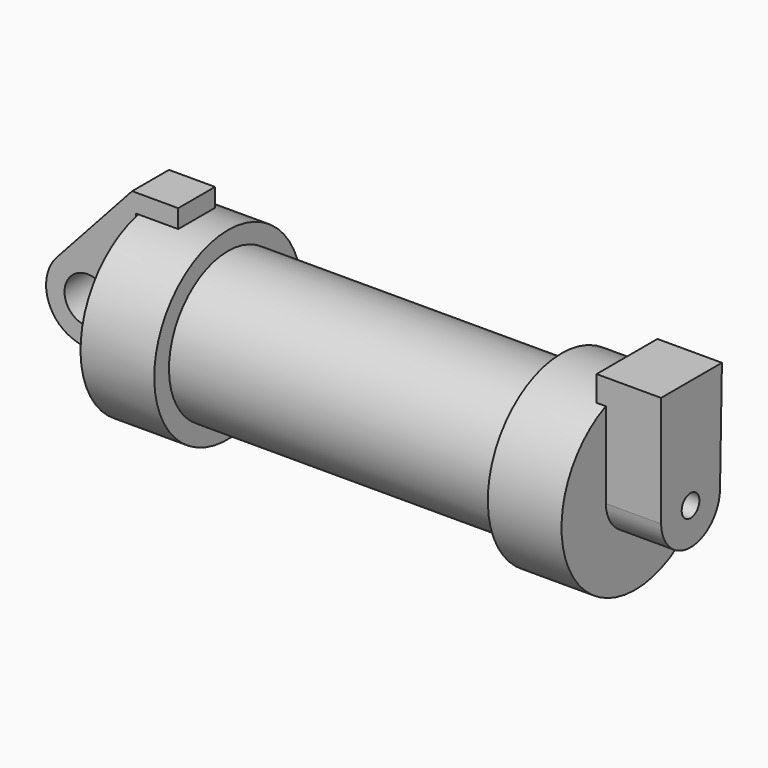
from build123d import *

# Parameters (mm, degrees)
F0_W          = 5.842
F0_H          = 12.7
F0_R          = 3.175
F2_DEPTH      = 3.175
F3_R          = 1.524
F4_DEPTH      = 7.62
F4_DEPTH_BACK = 1.27


with BuildPart() as f1:
    # F0 (on Front) → F1 (revolve)
    with BuildSketch(Plane.XZ):
        with Locations((2.921, 6.35)):
            Rectangle(F0_W, F0_H)
        Polygon((5.842, 12.7), (5.842, 0), (66.294, 0), (66.294, 12.7), (56.134, 12.7), (56.134, 10.16), (10.16, 10.16), (10.16, 12.7), align=None)
    revolve(axis=Axis((33.147, 0, 0), (-1, 0, 0)))

    # F3 (on face) → F4 (join, two sides)
    with BuildSketch(Plane.YZ.offset(66.294)) as f4_sk:
        with BuildLine():
            Line((-5.0772309735, 0.1677070124), (-5.0772309735, -0.1677070124))
            ThreePointArc((-5.0772309735, -0.1677070124), (0.0289763613, -5.0799173586), (5.0788137641, -0.1097759081))
            ThreePointArc((5.0788137641, -0.1097759081), (5.0797034324, -0.0548911586), (5.08, 0))
            ThreePointArc((5.08, 0), (0.0838649353, 5.0793076962), (-5.0772309735, 0.1677070124))
        make_face()
        Circle(F3_R, mode=Mode.SUBTRACT)
        with BuildLine():
            ThreePointArc((5.08, 0), (5.0797034324, -0.0548911586), (5.0788137641, -0.1097759081))
            Line((5.0788137641, -0.1097759081), (5.3303419683, 11.5272483491))
            ThreePointArc((5.3303419683, 11.5272483491), (0.1387383567, 12.6992421691), (-5.0772309735, 11.6409503754))
            Line((-5.0772309735, 11.6409503754), (-5.0772309735, 0.1677070124))
            ThreePointArc((-5.0772309735, 0.1677070124), (0.0838649353, 5.0793076962), (5.08, 0))
        make_face()
        with BuildLine():
            ThreePointArc((-5.0772309735, 11.6409503754), (0.1387383567, 12.6992421691), (5.3303419683, 11.5272483491))
            Line((5.3303419683, 11.5272483491), (5.408218408, 15.1302240919))
            Line((5.408218408, 15.1302240919), (-5.0772309735, 15.1302240919))
            Line((-5.0772309735, 15.1302240919), (-5.0772309735, 11.6409503754))
        make_face()
    extrude(amount=F4_DEPTH)
    extrude(f4_sk.sketch, amount=-F4_DEPTH_BACK)


with BuildPart() as f2:
    # F0 (on Front) → F2 (new body, symmetric)
    with BuildSketch(Plane.XZ):
        with BuildLine():
            Line((-0.9398, 0), (0, 0))
            Line((0, 0), (0, 12.7))
            Line((0, 12.7), (5.842, 12.7))
            Line((5.842, 12.7), (5.842, 15.24))
            Line((5.842, 15.24), (-0.508, 15.24))
            Line((-0.508, 15.24), (-10.8806298187, 3.8475430269))
            ThreePointArc((-10.8806298187, 3.8475430269), (-4.5919612295, 5.3297205562), (-0.9398, 0))
        make_face()
        with BuildLine():
            ThreePointArc((-8.1826630726, -5.5069827884), (-3.1957909266, -4.5493385486), (-0.9398, 0))
            ThreePointArc((-0.9398, 0), (-4.5919612295, 5.3297205562), (-10.8806298187, 3.8475430269))
            ThreePointArc((-10.8806298187, 3.8475430269), (-12.1459778134, -1.5837270034), (-8.1826630726, -5.5069827884))
        make_face()
        with Locations((-6.6548, 0)):
            Circle(F0_R, mode=Mode.SUBTRACT)
        with BuildLine():
            Line((5.842, 0), (0, 0))
            Line((0, 0), (-0.9398, 0))
            ThreePointArc((-0.9398, 0), (-3.1957909266, -4.5493385486), (-8.1826630726, -5.5069827884))
            Line((-8.1826630726, -5.5069827884), (5.842, -9.398))
            Line((5.842, -9.398), (5.842, 0))
        make_face()
    extrude(amount=F2_DEPTH, both=True)


solid = Compound([f1.part, f2.part])
